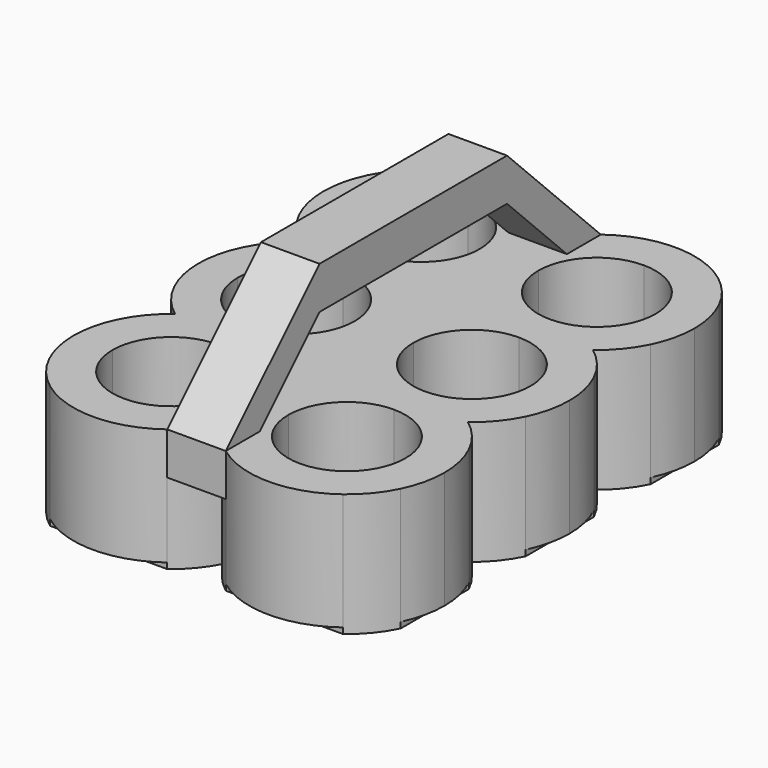
from build123d import *

# Parameters (mm, degrees)
F1_DEPTH = 25.4
F2_DEPTH = 1.27
F4_DEPTH = 6.35


with BuildPart() as f1:
    # F0 (on Top) → F1 (new body)
    with BuildSketch(Plane.XY):
        with BuildLine():
            Line((-2.1166666667, 33.8666666667), (-6.35, 33.8666666667))
            ThreePointArc((-6.35, 33.8666666667), (-10.0697438789, 24.8864105456), (-19.05, 21.1666666667))
            ThreePointArc((-19.05, 21.1666666667), (-12.356512286, 20.0804631421), (-6.35, 16.9333333333))
            ThreePointArc((-6.35, 16.9333333333), (-2.7139944723, 20.4069972362), (0, 24.6403305695))
            ThreePointArc((0, 24.6403305695), (-1.5807146965, 29.1336561143), (-2.1166666667, 33.8666666667))
        make_face()
        with BuildLine():
            ThreePointArc((-19.05, 46.5666666667), (-10.0697438789, 42.8469227877), (-6.35, 33.8666666667))
            Line((-6.35, 33.8666666667), (-2.1166666667, 33.8666666667))
            ThreePointArc((-2.1166666667, 33.8666666667), (-1.5807146965, 38.5996772191), (0, 43.0930027638))
            ThreePointArc((0, 43.0930027638), (-2.7139944723, 47.3263360972), (-6.35, 50.8))
            Line((-6.35, 50.8), (-19.05, 50.8))
            Line((-19.05, 50.8), (-19.05, 46.5666666667))
        make_face()
        with BuildLine():
            ThreePointArc((-31.75, 33.8666666667), (-28.0302561211, 42.8469227877), (-19.05, 46.5666666667))
            Line((-19.05, 46.5666666667), (-19.05, 50.8))
            Line((-19.05, 50.8), (-31.75, 50.8))
            ThreePointArc((-31.75, 50.8), (-35.3860055277, 47.3263360972), (-38.1, 43.0930027638))
            Line((-38.1, 43.0930027638), (-38.1, 33.8666666667))
            Line((-38.1, 33.8666666667), (-31.75, 33.8666666667))
        make_face()
        with BuildLine():
            ThreePointArc((-31.75, 16.9333333333), (-25.743487714, 20.0804631421), (-19.05, 21.1666666667))
            ThreePointArc((-19.05, 21.1666666667), (-28.0302561211, 24.8864105456), (-31.75, 33.8666666667))
            Line((-31.75, 33.8666666667), (-38.1, 33.8666666667))
            Line((-38.1, 33.8666666667), (-38.1, 24.6403305695))
            ThreePointArc((-38.1, 24.6403305695), (-35.3860055277, 20.4069972362), (-31.75, 16.9333333333))
        make_face()
        with BuildLine():
            ThreePointArc((-6.35, 16.9333333333), (-12.356512286, 20.0804631421), (-19.05, 21.1666666667))
            Line((-19.05, 21.1666666667), (-19.05, 16.9333333333))
            Line((-19.05, 16.9333333333), (-6.35, 16.9333333333))
        make_face()
        with BuildLine():
            Line((-19.05, 16.9333333333), (-19.05, 21.1666666667))
            ThreePointArc((-19.05, 21.1666666667), (-25.743487714, 20.0804631421), (-31.75, 16.9333333333))
            Line((-31.75, 16.9333333333), (-19.05, 16.9333333333))
        make_face()
        with BuildLine():
            ThreePointArc((0, 43.0930027638), (-1.5807146965, 38.5996772191), (-2.1166666667, 33.8666666667))
            Line((-2.1166666667, 33.8666666667), (0, 33.8666666667))
            Line((0, 33.8666666667), (0, 43.0930027638))
        make_face()
        with BuildLine():
            Line((0, 33.8666666667), (-2.1166666667, 33.8666666667))
            ThreePointArc((-2.1166666667, 33.8666666667), (-1.5807146965, 29.1336561143), (0, 24.6403305695))
            Line((0, 24.6403305695), (0, 33.8666666667))
        make_face()
        with BuildLine():
            Line((-31.75, 50.8), (-19.05, 50.8))
            Line((-19.05, 50.8), (-6.35, 50.8))
            ThreePointArc((-6.35, 50.8), (-19.05, 55.0333333333), (-31.75, 50.8))
        make_face()
        with BuildLine():
            Line((-6.35, 16.9333333333), (-19.05, 16.9333333333))
            Line((-19.05, 16.9333333333), (-19.05, 12.7))
            ThreePointArc((-19.0500000333, 12.7), (-12.3565123018, 13.7862035193), (-6.35, 16.9333333333))
        make_face()
        with BuildLine():
            Line((-19.05, 12.7), (-19.05, 16.9333333333))
            Line((-19.05, 16.9333333333), (-31.75, 16.9333333333))
            ThreePointArc((-31.75, 16.9333333333), (-25.7434877298, 13.7862035299), (-19.0500000333, 12.7))
        make_face()
        with BuildLine():
            ThreePointArc((0, 24.6403305695), (-2.7139944723, 20.4069972362), (-6.35, 16.9333333333))
            Line((-6.35, 16.9333333333), (0, 16.9333333333))
            Line((0, 16.9333333333), (0, 24.6403305695))
        make_face()
        with BuildLine():
            Line((0, 16.9333333333), (-6.35, 16.9333333333))
            ThreePointArc((-6.35, 16.9333333333), (-2.7139944723, 13.4596694305), (0, 9.2263360972))
            Line((0, 9.2263360972), (0, 16.9333333333))
        make_face()
        with BuildLine():
            ThreePointArc((0, 9.2263360972), (-2.7139944723, 13.4596694305), (-6.35, 16.9333333333))
            ThreePointArc((-6.35, 16.9333333333), (-12.3565123018, 13.7862035193), (-19.0500000333, 12.7))
            ThreePointArc((-19.0500000333, 12.7), (-10.0697438907, 8.9802561328), (-6.35, 0))
            Line((-6.35, 0), (-2.1166666667, 0))
            ThreePointArc((-2.1166666667, 0), (-1.5807146965, 4.7330105524), (0, 9.2263360972))
        make_face()
        with BuildLine():
            ThreePointArc((-19.0500000333, 12.7), (-25.7434877298, 13.7862035299), (-31.75, 16.9333333333))
            ThreePointArc((-31.75, 16.9333333333), (-35.3860055277, 13.4596694305), (-38.1, 9.2263360972))
            Line((-38.1, 9.2263360972), (-38.1, 0))
            Line((-38.1, 0), (-31.75, 0))
            ThreePointArc((-31.75, 0), (-28.0302561328, 8.9802561093), (-19.0500000333, 12.7))
        make_face()
        with BuildLine():
            Line((2.1166666667, 33.8666666667), (0, 33.8666666667))
            Line((0, 33.8666666667), (0, 24.6403305695))
            ThreePointArc((0, 24.6403305695), (1.5807146965, 29.1336561143), (2.1166666667, 33.8666666667))
        make_face()
        with BuildLine():
            Line((0, 43.0930027638), (0, 33.8666666667))
            Line((0, 33.8666666667), (2.1166666667, 33.8666666667))
            ThreePointArc((2.1166666667, 33.8666666667), (1.5807146965, 38.5996772191), (0, 43.0930027638))
        make_face()
        with BuildLine():
            ThreePointArc((6.35, 50.8), (2.7139944723, 47.3263360972), (0, 43.0930027638))
            ThreePointArc((0, 43.0930027638), (1.5807146965, 38.5996772191), (2.1166666667, 33.8666666667))
            Line((2.1166666667, 33.8666666667), (6.35, 33.8666666667))
            ThreePointArc((6.35, 33.8666666667), (10.0697438789, 42.8469227877), (19.05, 46.5666666667))
            Line((19.05, 46.5666666667), (19.05, 50.8))
            Line((19.05, 50.8), (6.35, 50.8))
        make_face()
        with BuildLine():
            ThreePointArc((6.35, 16.9333333333), (2.7139944723, 20.4069972362), (0, 24.6403305695))
            Line((0, 24.6403305695), (0, 16.9333333333))
            Line((0, 16.9333333333), (6.35, 16.9333333333))
        make_face()
        with BuildLine():
            ThreePointArc((2.1166666667, 33.8666666667), (1.5807146965, 29.1336561143), (0, 24.6403305695))
            ThreePointArc((0, 24.6403305695), (2.7139944723, 20.4069972362), (6.35, 16.9333333333))
            ThreePointArc((6.35, 16.9333333333), (12.356512286, 20.0804631421), (19.05, 21.1666666667))
            ThreePointArc((19.05, 21.1666666667), (10.0697438789, 24.8864105456), (6.35, 33.8666666667))
            Line((6.35, 33.8666666667), (2.1166666667, 33.8666666667))
        make_face()
        with BuildLine():
            Line((-38.1, 24.6403305695), (-38.1, 33.8666666667))
            Line((-38.1, 33.8666666667), (-38.1, 43.0930027638))
            ThreePointArc((-38.1, 43.0930027638), (-40.2166666667, 33.8666666667), (-38.1, 24.6403305695))
        make_face()
        with BuildLine():
            Line((6.35, 16.9333333333), (0, 16.9333333333))
            Line((0, 16.9333333333), (0, 9.2263360972))
            ThreePointArc((0, 9.2263360972), (2.7139944723, 13.4596694305), (6.35, 16.9333333333))
        make_face()
        with BuildLine():
            ThreePointArc((2.1166666667, 0), (1.5807146965, 4.7330105524), (0, 9.2263360972))
            Line((0, 9.2263360972), (0, 0))
            Line((0, 0), (2.1166666667, 0))
        make_face()
        with BuildLine():
            ThreePointArc((6.35, 16.9333333333), (2.7139944723, 13.4596694305), (0, 9.2263360972))
            ThreePointArc((0, 9.2263360972), (1.5807146965, 4.7330105524), (2.1166666667, 0))
            Line((2.1166666667, 0), (6.35, 0))
            ThreePointArc((6.35, 0), (10.0697438672, 8.9802561093), (19.0499999667, 12.7))
            ThreePointArc((19.0499999667, 12.7), (12.3565122702, 13.7862035299), (6.35, 16.9333333333))
        make_face()
        with BuildLine():
            Line((0, 0), (0, 9.2263360972))
            ThreePointArc((0, 9.2263360972), (-1.5807146965, 4.7330105524), (-2.1166666667, 0))
            Line((-2.1166666667, 0), (0, 0))
        make_face()
        with BuildLine():
            Line((-38.1, 0), (-38.1, 9.2263360972))
            ThreePointArc((-38.1, 9.2263360972), (-40.2166666667, 0), (-38.1, -9.2263360972))
            Line((-38.1, -9.2263360972), (-38.1, 0))
        make_face()
        with BuildLine():
            ThreePointArc((31.75, 50.8), (19.05, 55.0333333333), (6.35, 50.8))
            Line((6.35, 50.8), (19.05, 50.8))
            Line((19.05, 50.8), (31.75, 50.8))
        make_face()
        with BuildLine():
            ThreePointArc((19.05, 21.1666666667), (12.356512286, 20.0804631421), (6.35, 16.9333333333))
            Line((6.35, 16.9333333333), (19.05, 16.9333333333))
            Line((19.05, 16.9333333333), (19.05, 21.1666666667))
        make_face()
        with BuildLine():
            Line((19.05, 16.9333333333), (6.35, 16.9333333333))
            ThreePointArc((6.35, 16.9333333333), (12.3565122702, 13.7862035299), (19.0499999667, 12.7))
            Line((19.05, 12.7), (19.05, 16.9333333333))
        make_face()
        with BuildLine():
            Line((-2.1166666667, 0), (-6.35, 0))
            ThreePointArc((-6.35, 0), (-10.0697438789, -8.9802561211), (-19.05, -12.7))
            ThreePointArc((-19.05, -12.7), (-12.356512286, -13.7862035246), (-6.35, -16.9333333333))
            ThreePointArc((-6.35, -16.9333333333), (-2.7139944723, -13.4596694305), (0, -9.2263360972))
            ThreePointArc((0, -9.2263360972), (-1.5807146965, -4.7330105524), (-2.1166666667, 0))
        make_face()
        with BuildLine():
            ThreePointArc((-19.05, -12.7), (-28.0302561211, -8.9802561211), (-31.75, 0))
            Line((-31.75, 0), (-38.1, 0))
            Line((-38.1, 0), (-38.1, -9.2263360972))
            ThreePointArc((-38.1, -9.2263360972), (-35.3860055277, -13.4596694305), (-31.75, -16.9333333333))
            ThreePointArc((-31.75, -16.9333333333), (-25.743487714, -13.7862035246), (-19.05, -12.7))
        make_face()
        with BuildLine():
            Line((2.1166666667, 0), (0, 0))
            Line((0, 0), (0, -9.2263360972))
            ThreePointArc((0, -9.2263360972), (1.5807146965, -4.7330105524), (2.1166666667, 0))
        make_face()
        with BuildLine():
            Line((0, -9.2263360972), (0, 0))
            Line((0, 0), (-2.1166666667, 0))
            ThreePointArc((-2.1166666667, 0), (-1.5807146965, -4.7330105524), (0, -9.2263360972))
        make_face()
        with BuildLine():
            Line((6.35, 0), (2.1166666667, 0))
            ThreePointArc((2.1166666667, 0), (1.5807146965, -4.7330105524), (0, -9.2263360972))
            ThreePointArc((0, -9.2263360972), (2.7139944723, -13.4596694305), (6.35, -16.9333333333))
            ThreePointArc((6.35, -16.9333333333), (12.356512286, -13.7862035246), (19.05, -12.7))
            ThreePointArc((19.05, -12.7), (10.0697438789, -8.9802561211), (6.35, 0))
        make_face()
        with BuildLine():
            Line((31.75, 50.8), (19.05, 50.8))
            Line((19.05, 50.8), (19.05, 46.5666666667))
            ThreePointArc((19.05, 46.5666666667), (28.0302561211, 42.8469227877), (31.75, 33.8666666667))
            Line((31.75, 33.8666666667), (38.1, 33.8666666667))
            Line((38.1, 33.8666666667), (38.1, 43.0930027638))
            ThreePointArc((38.1, 43.0930027638), (35.3860055277, 47.3263360972), (31.75, 50.8))
        make_face()
        with BuildLine():
            Line((31.75, 16.9333333333), (19.05, 16.9333333333))
            Line((19.05, 16.9333333333), (19.05, 12.7))
            ThreePointArc((19.0499999667, 12.7), (25.7434876982, 13.7862035193), (31.75, 16.9333333333))
        make_face()
        with BuildLine():
            Line((19.05, 21.1666666667), (19.05, 16.9333333333))
            Line((19.05, 16.9333333333), (31.75, 16.9333333333))
            ThreePointArc((31.75, 16.9333333333), (25.743487714, 20.0804631421), (19.05, 21.1666666667))
        make_face()
        with BuildLine():
            ThreePointArc((31.75, 33.8666666667), (28.0302561211, 24.8864105456), (19.05, 21.1666666667))
            ThreePointArc((19.05, 21.1666666667), (25.743487714, 20.0804631421), (31.75, 16.9333333333))
            ThreePointArc((31.75, 16.9333333333), (35.3860055277, 20.4069972362), (38.1, 24.6403305695))
            Line((38.1, 24.6403305695), (38.1, 33.8666666667))
            Line((38.1, 33.8666666667), (31.75, 33.8666666667))
        make_face()
        with BuildLine():
            ThreePointArc((31.75, 16.9333333333), (25.7434876982, 13.7862035193), (19.0499999667, 12.7))
            ThreePointArc((19.0499999667, 12.7), (28.0302561093, 8.9802561328), (31.75, 0))
            Line((31.75, 0), (38.1, 0))
            Line((38.1, 0), (38.1, 9.2263360972))
            ThreePointArc((38.1, 9.2263360972), (35.3860055277, 13.4596694305), (31.75, 16.9333333333))
        make_face()
        with BuildLine():
            ThreePointArc((-6.35, -16.9333333333), (-12.356512286, -13.7862035246), (-19.05, -12.7))
            Line((-19.05, -12.7), (-19.05, -16.9333333333))
            Line((-19.05, -16.9333333333), (-6.35, -16.9333333333))
        make_face()
        with BuildLine():
            Line((-19.05, -16.9333333333), (-19.05, -12.7))
            ThreePointArc((-19.05, -12.7), (-25.743487714, -13.7862035246), (-31.75, -16.9333333333))
            Line((-31.75, -16.9333333333), (-19.05, -16.9333333333))
        make_face()
        with BuildLine():
            ThreePointArc((6.35, -16.9333333333), (2.7139944723, -13.4596694305), (0, -9.2263360972))
            Line((0, -9.2263360972), (0, -16.9333333333))
            Line((0, -16.9333333333), (6.35, -16.9333333333))
        make_face()
        with BuildLine():
            Line((0, -16.9333333333), (0, -9.2263360972))
            ThreePointArc((0, -9.2263360972), (-2.7139944723, -13.4596694305), (-6.35, -16.9333333333))
            Line((-6.35, -16.9333333333), (0, -16.9333333333))
        make_face()
        with BuildLine():
            Line((-19.05, -16.9333333333), (-31.75, -16.9333333333))
            ThreePointArc((-31.75, -16.9333333333), (-25.7434877142, -20.080463142), (-19.0500000004, -21.1666666667))
            Line((-19.05, -21.1666666667), (-19.05, -16.9333333333))
        make_face()
        with BuildLine():
            ThreePointArc((-19.0500000004, -21.1666666667), (-25.7434877142, -20.080463142), (-31.75, -16.9333333333))
            ThreePointArc((-31.75, -16.9333333333), (-35.3860055277, -20.4069972362), (-38.1, -24.6403305695))
            Line((-38.1, -24.6403305695), (-38.1, -33.8666666667))
            Line((-38.1, -33.8666666667), (-31.75, -33.8666666667))
            ThreePointArc((-31.75, -33.8666666667), (-28.0302561212, -24.8864105457), (-19.0500000004, -21.1666666667))
        make_face()
        with BuildLine():
            ThreePointArc((40.2166666667, 33.8666666667), (39.6807146965, 38.5996772191), (38.1, 43.0930027638))
            Line((38.1, 43.0930027638), (38.1, 33.8666666667))
            Line((38.1, 33.8666666667), (38.1, 24.6403305695))
            ThreePointArc((38.1, 24.6403305695), (39.6807146965, 29.1336561143), (40.2166666667, 33.8666666667))
        make_face()
        with BuildLine():
            Line((38.1, 0), (31.75, 0))
            ThreePointArc((31.75, 0), (28.0302561211, -8.9802561211), (19.05, -12.7))
            ThreePointArc((19.05, -12.7), (25.743487714, -13.7862035246), (31.75, -16.9333333333))
            ThreePointArc((31.75, -16.9333333333), (35.3860055277, -13.4596694305), (38.1, -9.2263360972))
            Line((38.1, -9.2263360972), (38.1, 0))
        make_face()
        with BuildLine():
            Line((-6.35, -16.9333333333), (-19.05, -16.9333333333))
            Line((-19.05, -16.9333333333), (-19.05, -21.1666666667))
            ThreePointArc((-19.0500000004, -21.1666666667), (-12.3565122862, -20.0804631421), (-6.35, -16.9333333333))
        make_face()
        with BuildLine():
            ThreePointArc((0, -24.6403305695), (-2.7139944723, -20.4069972362), (-6.35, -16.9333333333))
            ThreePointArc((-6.35, -16.9333333333), (-12.3565122862, -20.0804631421), (-19.0500000004, -21.1666666667))
            ThreePointArc((-19.0500000004, -21.1666666667), (-10.0697438791, -24.8864105455), (-6.35, -33.8666666667))
            Line((-6.35, -33.8666666667), (-2.1166666667, -33.8666666667))
            ThreePointArc((-2.1166666667, -33.8666666667), (-1.5807146965, -29.1336561143), (0, -24.6403305695))
        make_face()
        with BuildLine():
            Line((0, -16.9333333333), (-6.35, -16.9333333333))
            ThreePointArc((-6.35, -16.9333333333), (-2.7139944723, -20.4069972362), (0, -24.6403305695))
            Line((0, -24.6403305695), (0, -16.9333333333))
        make_face()
        with BuildLine():
            Line((6.35, -16.9333333333), (0, -16.9333333333))
            Line((0, -16.9333333333), (0, -24.6403305695))
            ThreePointArc((0, -24.6403305695), (2.7139944723, -20.4069972362), (6.35, -16.9333333333))
        make_face()
        with BuildLine():
            ThreePointArc((19.05, -12.7), (12.356512286, -13.7862035246), (6.35, -16.9333333333))
            Line((6.35, -16.9333333333), (19.05, -16.9333333333))
            Line((19.05, -16.9333333333), (19.05, -12.7))
        make_face()
        with BuildLine():
            Line((19.05, -16.9333333333), (6.35, -16.9333333333))
            ThreePointArc((6.35, -16.9333333333), (12.3565122858, -20.080463142), (19.0499999996, -21.1666666667))
            Line((19.05, -21.1666666667), (19.05, -16.9333333333))
        make_face()
        with BuildLine():
            ThreePointArc((19.0499999996, -21.1666666667), (12.3565122858, -20.080463142), (6.35, -16.9333333333))
            ThreePointArc((6.35, -16.9333333333), (2.7139944723, -20.4069972362), (0, -24.6403305695))
            ThreePointArc((0, -24.6403305695), (1.5807146965, -29.1336561143), (2.1166666667, -33.8666666667))
            Line((2.1166666667, -33.8666666667), (6.35, -33.8666666667))
            ThreePointArc((6.35, -33.8666666667), (10.0697438788, -24.8864105457), (19.0499999996, -21.1666666667))
        make_face()
        with BuildLine():
            ThreePointArc((31.75, -16.9333333333), (25.743487714, -13.7862035246), (19.05, -12.7))
            Line((19.05, -12.7), (19.05, -16.9333333333))
            Line((19.05, -16.9333333333), (31.75, -16.9333333333))
        make_face()
        with BuildLine():
            Line((-38.1, -33.8666666667), (-38.1, -24.6403305695))
            ThreePointArc((-38.1, -24.6403305695), (-40.2166666667, -33.8666666667), (-38.1, -43.0930027638))
            Line((-38.1, -43.0930027638), (-38.1, -33.8666666667))
        make_face()
        with BuildLine():
            ThreePointArc((40.2166666667, 0), (39.6807146965, 4.7330105524), (38.1, 9.2263360972))
            Line((38.1, 9.2263360972), (38.1, 0))
            Line((38.1, 0), (38.1, -9.2263360972))
            ThreePointArc((38.1, -9.2263360972), (39.6807146965, -4.7330105524), (40.2166666667, 0))
        make_face()
        with BuildLine():
            ThreePointArc((2.1166666667, -33.8666666667), (1.5807146965, -29.1336561143), (0, -24.6403305695))
            Line((0, -24.6403305695), (0, -33.8666666667))
            Line((0, -33.8666666667), (2.1166666667, -33.8666666667))
        make_face()
        with BuildLine():
            Line((0, -33.8666666667), (0, -24.6403305695))
            ThreePointArc((0, -24.6403305695), (-1.5807146965, -29.1336561143), (-2.1166666667, -33.8666666667))
            Line((-2.1166666667, -33.8666666667), (0, -33.8666666667))
        make_face()
        with BuildLine():
            Line((31.75, -16.9333333333), (19.05, -16.9333333333))
            Line((19.05, -16.9333333333), (19.05, -21.1666666667))
            ThreePointArc((19.0499999996, -21.1666666667), (25.7434877138, -20.0804631421), (31.75, -16.9333333333))
        make_face()
        with BuildLine():
            ThreePointArc((31.75, -16.9333333333), (25.7434877138, -20.0804631421), (19.0499999996, -21.1666666667))
            ThreePointArc((19.0499999996, -21.1666666667), (28.0302561209, -24.8864105455), (31.75, -33.8666666667))
            Line((31.75, -33.8666666667), (38.1, -33.8666666667))
            Line((38.1, -33.8666666667), (38.1, -24.6403305695))
            ThreePointArc((38.1, -24.6403305695), (35.3860055277, -20.4069972362), (31.75, -16.9333333333))
        make_face()
        with BuildLine():
            Line((-31.75, -33.8666666667), (-38.1, -33.8666666667))
            Line((-38.1, -33.8666666667), (-38.1, -43.0930027638))
            ThreePointArc((-38.1, -43.0930027638), (-35.3860055276, -47.3263360972), (-31.75, -50.8))
            Line((-31.75, -50.8), (-19.05, -50.8))
            Line((-19.05, -50.8), (-19.05, -46.5666666667))
            ThreePointArc((-19.05, -46.5666666667), (-28.0302561211, -42.8469227877), (-31.75, -33.8666666667))
        make_face()
        with BuildLine():
            Line((-2.1166666667, -33.8666666667), (-6.35, -33.8666666667))
            ThreePointArc((-6.35, -33.8666666667), (-10.0697438789, -42.8469227877), (-19.05, -46.5666666667))
            Line((-19.05, -46.5666666667), (-19.05, -50.8))
            Line((-19.05, -50.8), (-6.35, -50.8))
            ThreePointArc((-6.35, -50.8), (-2.7139944724, -47.3263360971), (0, -43.0930027638))
            ThreePointArc((0, -43.0930027638), (-1.5807146965, -38.599677219), (-2.1166666667, -33.8666666667))
        make_face()
        with BuildLine():
            Line((2.1166666667, -33.8666666667), (0, -33.8666666667))
            Line((0, -33.8666666667), (0, -43.0930027638))
            ThreePointArc((0, -43.0930027638), (1.5807146965, -38.599677219), (2.1166666667, -33.8666666667))
        make_face()
        with BuildLine():
            Line((0, -43.0930027638), (0, -33.8666666667))
            Line((0, -33.8666666667), (-2.1166666667, -33.8666666667))
            ThreePointArc((-2.1166666667, -33.8666666667), (-1.5807146965, -38.599677219), (0, -43.0930027638))
        make_face()
        with BuildLine():
            Line((6.35, -33.8666666667), (2.1166666667, -33.8666666667))
            ThreePointArc((2.1166666667, -33.8666666667), (1.5807146965, -38.599677219), (0, -43.0930027638))
            ThreePointArc((0, -43.0930027638), (2.7139944724, -47.3263360972), (6.35, -50.8))
            Line((6.35, -50.8), (19.05, -50.8))
            Line((19.05, -50.8), (19.05, -46.5666666667))
            ThreePointArc((19.05, -46.5666666667), (10.0697438789, -42.8469227877), (6.35, -33.8666666667))
        make_face()
        with BuildLine():
            Line((38.1, -33.8666666667), (31.75, -33.8666666667))
            ThreePointArc((31.75, -33.8666666667), (28.0302561211, -42.8469227877), (19.05, -46.5666666667))
            Line((19.05, -46.5666666667), (19.05, -50.8))
            Line((19.05, -50.8), (31.75, -50.8))
            ThreePointArc((31.75, -50.8), (35.3860055276, -47.3263360971), (38.1, -43.0930027638))
            Line((38.1, -43.0930027638), (38.1, -33.8666666667))
        make_face()
        with BuildLine():
            ThreePointArc((40.2166666667, -33.8666666667), (39.6807146965, -29.1336561143), (38.1, -24.6403305695))
            Line((38.1, -24.6403305695), (38.1, -33.8666666667))
            Line((38.1, -33.8666666667), (38.1, -43.0930027638))
            ThreePointArc((38.1, -43.0930027638), (39.6807146965, -38.599677219), (40.2166666667, -33.8666666667))
        make_face()
        with BuildLine():
            Line((-19.05, -50.8), (-31.75, -50.8))
            ThreePointArc((-31.75, -50.8), (-19.05, -55.0333333333), (-6.35, -50.8))
            Line((-6.35, -50.8), (-19.05, -50.8))
        make_face()
        with BuildLine():
            Line((19.05, -50.8), (6.35, -50.8))
            ThreePointArc((6.35, -50.8), (19.05, -55.0333333333), (31.75, -50.8))
            Line((31.75, -50.8), (19.05, -50.8))
        make_face()
    extrude(amount=F1_DEPTH)

    # F0 (on Top) → F2 (join, symmetric)
    with BuildSketch(Plane.XY):
        with BuildLine():
            Line((-19.05, 33.8666666667), (-19.05, 46.5666666667))
            ThreePointArc((-19.05, 46.5666666667), (-28.0302561211, 42.8469227877), (-31.75, 33.8666666667))
            Line((-31.75, 33.8666666667), (-19.05, 33.8666666667))
        make_face()
        with BuildLine():
            Line((-19.05, 33.8666666667), (-6.35, 33.8666666667))
            ThreePointArc((-6.35, 33.8666666667), (-10.0697438789, 42.8469227877), (-19.05, 46.5666666667))
            Line((-19.05, 46.5666666667), (-19.05, 33.8666666667))
        make_face()
        with BuildLine():
            ThreePointArc((-31.75, 33.8666666667), (-28.0302561211, 24.8864105456), (-19.05, 21.1666666667))
            Line((-19.05, 21.1666666667), (-19.05, 33.8666666667))
            Line((-19.05, 33.8666666667), (-31.75, 33.8666666667))
        make_face()
        with BuildLine():
            ThreePointArc((-19.05, 21.1666666667), (-10.0697438789, 24.8864105456), (-6.35, 33.8666666667))
            Line((-6.35, 33.8666666667), (-19.05, 33.8666666667))
            Line((-19.05, 33.8666666667), (-19.05, 21.1666666667))
        make_face()
        with BuildLine():
            ThreePointArc((19.05, 46.5666666667), (10.0697438789, 42.8469227877), (6.35, 33.8666666667))
            Line((6.35, 33.8666666667), (19.05, 33.8666666667))
            Line((19.05, 33.8666666667), (19.05, 46.5666666667))
        make_face()
        with BuildLine():
            ThreePointArc((31.75, 33.8666666667), (28.0302561211, 42.8469227877), (19.05, 46.5666666667))
            Line((19.05, 46.5666666667), (19.05, 33.8666666667))
            Line((19.05, 33.8666666667), (31.75, 33.8666666667))
        make_face()
        with BuildLine():
            Line((19.05, 33.8666666667), (19.05, 21.1666666667))
            ThreePointArc((19.05, 21.1666666667), (28.0302561211, 24.8864105456), (31.75, 33.8666666667))
            Line((31.75, 33.8666666667), (19.05, 33.8666666667))
        make_face()
        with BuildLine():
            Line((19.05, 33.8666666667), (6.35, 33.8666666667))
            ThreePointArc((6.35, 33.8666666667), (10.0697438789, 24.8864105456), (19.05, 21.1666666667))
            Line((19.05, 21.1666666667), (19.05, 33.8666666667))
        make_face()
        with BuildLine():
            Line((-19.05, 0), (-19.05, 12.7))
            ThreePointArc((-19.0500000333, 12.7), (-28.0302561328, 8.9802561093), (-31.75, 0))
            Line((-31.75, 0), (-19.05, 0))
        make_face()
        with BuildLine():
            ThreePointArc((-6.35, 0), (-10.0697438907, 8.9802561328), (-19.0500000333, 12.7))
            Line((-19.05, 12.7), (-19.05, 0))
            Line((-19.05, 0), (-6.35, 0))
        make_face()
        with BuildLine():
            Line((-19.05, 0), (-31.75, 0))
            ThreePointArc((-31.75, 0), (-28.0302561211, -8.9802561211), (-19.05, -12.7))
            Line((-19.05, -12.7), (-19.05, 0))
        make_face()
        with BuildLine():
            ThreePointArc((-19.05, -12.7), (-10.0697438789, -8.9802561211), (-6.35, 0))
            Line((-6.35, 0), (-19.05, 0))
            Line((-19.05, 0), (-19.05, -12.7))
        make_face()
        with BuildLine():
            Line((19.05, 0), (19.05, 12.7))
            ThreePointArc((19.0499999667, 12.7), (10.0697438672, 8.9802561093), (6.35, 0))
            Line((6.35, 0), (19.05, 0))
        make_face()
        with BuildLine():
            Line((19.05, 0), (6.35, 0))
            ThreePointArc((6.35, 0), (10.0697438789, -8.9802561211), (19.05, -12.7))
            Line((19.05, -12.7), (19.05, 0))
        make_face()
        with BuildLine():
            ThreePointArc((19.05, -12.7), (28.0302561211, -8.9802561211), (31.75, 0))
            Line((31.75, 0), (19.05, 0))
            Line((19.05, 0), (19.05, -12.7))
        make_face()
        with BuildLine():
            ThreePointArc((31.75, 0), (28.0302561093, 8.9802561328), (19.0499999667, 12.7))
            Line((19.05, 12.7), (19.05, 0))
            Line((19.05, 0), (31.75, 0))
        make_face()
        with BuildLine():
            ThreePointArc((-6.35, -33.8666666667), (-10.0697438791, -24.8864105455), (-19.0500000004, -21.1666666667))
            Line((-19.05, -21.1666666667), (-19.05, -33.8666666667))
            Line((-19.05, -33.8666666667), (-6.35, -33.8666666667))
        make_face()
        with BuildLine():
            Line((-19.05, -33.8666666667), (-19.05, -21.1666666667))
            ThreePointArc((-19.0500000004, -21.1666666667), (-28.0302561212, -24.8864105457), (-31.75, -33.8666666667))
            Line((-31.75, -33.8666666667), (-19.05, -33.8666666667))
        make_face()
        with BuildLine():
            Line((-19.05, -33.8666666667), (-31.75, -33.8666666667))
            ThreePointArc((-31.75, -33.8666666667), (-28.0302561211, -42.8469227877), (-19.05, -46.5666666667))
            Line((-19.05, -46.5666666667), (-19.05, -33.8666666667))
        make_face()
        with BuildLine():
            ThreePointArc((-19.05, -46.5666666667), (-10.0697438789, -42.8469227877), (-6.35, -33.8666666667))
            Line((-6.35, -33.8666666667), (-19.05, -33.8666666667))
            Line((-19.05, -33.8666666667), (-19.05, -46.5666666667))
        make_face()
        with BuildLine():
            Line((19.05, -33.8666666667), (19.05, -21.1666666667))
            ThreePointArc((19.0499999996, -21.1666666667), (10.0697438788, -24.8864105457), (6.35, -33.8666666667))
            Line((6.35, -33.8666666667), (19.05, -33.8666666667))
        make_face()
        with BuildLine():
            Line((19.05, -33.8666666667), (6.35, -33.8666666667))
            ThreePointArc((6.35, -33.8666666667), (10.0697438789, -42.8469227877), (19.05, -46.5666666667))
            Line((19.05, -46.5666666667), (19.05, -33.8666666667))
        make_face()
        with BuildLine():
            ThreePointArc((19.05, -46.5666666667), (28.0302561211, -42.8469227877), (31.75, -33.8666666667))
            Line((31.75, -33.8666666667), (19.05, -33.8666666667))
            Line((19.05, -33.8666666667), (19.05, -46.5666666667))
        make_face()
        with BuildLine():
            ThreePointArc((31.75, -33.8666666667), (28.0302561209, -24.8864105455), (19.0499999996, -21.1666666667))
            Line((19.05, -21.1666666667), (19.05, -33.8666666667))
            Line((19.05, -33.8666666667), (31.75, -33.8666666667))
        make_face()
        with BuildLine():
            Line((19.05, -16.9333333333), (6.35, -16.9333333333))
            ThreePointArc((6.35, -16.9333333333), (12.3565122858, -20.080463142), (19.0499999996, -21.1666666667))
            Line((19.05, -21.1666666667), (19.05, -16.9333333333))
        make_face()
        with BuildLine():
            Line((31.75, -16.9333333333), (19.05, -16.9333333333))
            Line((19.05, -16.9333333333), (19.05, -21.1666666667))
            ThreePointArc((19.0499999996, -21.1666666667), (25.7434877138, -20.0804631421), (31.75, -16.9333333333))
        make_face()
        with BuildLine():
            ThreePointArc((31.75, -16.9333333333), (25.743487714, -13.7862035246), (19.05, -12.7))
            Line((19.05, -12.7), (19.05, -16.9333333333))
            Line((19.05, -16.9333333333), (31.75, -16.9333333333))
        make_face()
        with BuildLine():
            ThreePointArc((19.05, -12.7), (12.356512286, -13.7862035246), (6.35, -16.9333333333))
            Line((6.35, -16.9333333333), (19.05, -16.9333333333))
            Line((19.05, -16.9333333333), (19.05, -12.7))
        make_face()
        with BuildLine():
            ThreePointArc((-6.35, -16.9333333333), (-12.356512286, -13.7862035246), (-19.05, -12.7))
            Line((-19.05, -12.7), (-19.05, -16.9333333333))
            Line((-19.05, -16.9333333333), (-6.35, -16.9333333333))
        make_face()
        with BuildLine():
            Line((-6.35, -16.9333333333), (-19.05, -16.9333333333))
            Line((-19.05, -16.9333333333), (-19.05, -21.1666666667))
            ThreePointArc((-19.0500000004, -21.1666666667), (-12.3565122862, -20.0804631421), (-6.35, -16.9333333333))
        make_face()
        with BuildLine():
            Line((-19.05, -16.9333333333), (-31.75, -16.9333333333))
            ThreePointArc((-31.75, -16.9333333333), (-25.7434877142, -20.080463142), (-19.0500000004, -21.1666666667))
            Line((-19.05, -21.1666666667), (-19.05, -16.9333333333))
        make_face()
        with BuildLine():
            Line((-19.05, -16.9333333333), (-19.05, -12.7))
            ThreePointArc((-19.05, -12.7), (-25.743487714, -13.7862035246), (-31.75, -16.9333333333))
            Line((-31.75, -16.9333333333), (-19.05, -16.9333333333))
        make_face()
        with BuildLine():
            Line((-19.05, 16.9333333333), (-19.05, 21.1666666667))
            ThreePointArc((-19.05, 21.1666666667), (-25.743487714, 20.0804631421), (-31.75, 16.9333333333))
            Line((-31.75, 16.9333333333), (-19.05, 16.9333333333))
        make_face()
        with BuildLine():
            Line((-19.05, 12.7), (-19.05, 16.9333333333))
            Line((-19.05, 16.9333333333), (-31.75, 16.9333333333))
            ThreePointArc((-31.75, 16.9333333333), (-25.7434877298, 13.7862035299), (-19.0500000333, 12.7))
        make_face()
        with BuildLine():
            Line((-6.35, 16.9333333333), (-19.05, 16.9333333333))
            Line((-19.05, 16.9333333333), (-19.05, 12.7))
            ThreePointArc((-19.0500000333, 12.7), (-12.3565123018, 13.7862035193), (-6.35, 16.9333333333))
        make_face()
        with BuildLine():
            ThreePointArc((-6.35, 16.9333333333), (-12.356512286, 20.0804631421), (-19.05, 21.1666666667))
            Line((-19.05, 21.1666666667), (-19.05, 16.9333333333))
            Line((-19.05, 16.9333333333), (-6.35, 16.9333333333))
        make_face()
        with BuildLine():
            ThreePointArc((19.05, 21.1666666667), (12.356512286, 20.0804631421), (6.35, 16.9333333333))
            Line((6.35, 16.9333333333), (19.05, 16.9333333333))
            Line((19.05, 16.9333333333), (19.05, 21.1666666667))
        make_face()
        with BuildLine():
            Line((19.05, 16.9333333333), (6.35, 16.9333333333))
            ThreePointArc((6.35, 16.9333333333), (12.3565122702, 13.7862035299), (19.0499999667, 12.7))
            Line((19.05, 12.7), (19.05, 16.9333333333))
        make_face()
        with BuildLine():
            Line((31.75, 16.9333333333), (19.05, 16.9333333333))
            Line((19.05, 16.9333333333), (19.05, 12.7))
            ThreePointArc((19.0499999667, 12.7), (25.7434876982, 13.7862035193), (31.75, 16.9333333333))
        make_face()
        with BuildLine():
            Line((19.05, 21.1666666667), (19.05, 16.9333333333))
            Line((19.05, 16.9333333333), (31.75, 16.9333333333))
            ThreePointArc((31.75, 16.9333333333), (25.743487714, 20.0804631421), (19.05, 21.1666666667))
        make_face()
        with BuildLine():
            Line((2.1166666667, 33.8666666667), (0, 33.8666666667))
            Line((0, 33.8666666667), (0, 24.6403305695))
            ThreePointArc((0, 24.6403305695), (1.5807146965, 29.1336561143), (2.1166666667, 33.8666666667))
        make_face()
        with BuildLine():
            Line((0, 33.8666666667), (-2.1166666667, 33.8666666667))
            ThreePointArc((-2.1166666667, 33.8666666667), (-1.5807146965, 29.1336561143), (0, 24.6403305695))
            Line((0, 24.6403305695), (0, 33.8666666667))
        make_face()
        with BuildLine():
            ThreePointArc((0, 43.0930027638), (-1.5807146965, 38.5996772191), (-2.1166666667, 33.8666666667))
            Line((-2.1166666667, 33.8666666667), (0, 33.8666666667))
            Line((0, 33.8666666667), (0, 43.0930027638))
        make_face()
        with BuildLine():
            Line((0, 43.0930027638), (0, 33.8666666667))
            Line((0, 33.8666666667), (2.1166666667, 33.8666666667))
            ThreePointArc((2.1166666667, 33.8666666667), (1.5807146965, 38.5996772191), (0, 43.0930027638))
        make_face()
        with BuildLine():
            ThreePointArc((-19.05, 46.5666666667), (-10.0697438789, 42.8469227877), (-6.35, 33.8666666667))
            Line((-6.35, 33.8666666667), (-2.1166666667, 33.8666666667))
            ThreePointArc((-2.1166666667, 33.8666666667), (-1.5807146965, 38.5996772191), (0, 43.0930027638))
            ThreePointArc((0, 43.0930027638), (-2.7139944723, 47.3263360972), (-6.35, 50.8))
            Line((-6.35, 50.8), (-19.05, 50.8))
            Line((-19.05, 50.8), (-19.05, 46.5666666667))
        make_face()
        with BuildLine():
            Line((-2.1166666667, 33.8666666667), (-6.35, 33.8666666667))
            ThreePointArc((-6.35, 33.8666666667), (-10.0697438789, 24.8864105456), (-19.05, 21.1666666667))
            ThreePointArc((-19.05, 21.1666666667), (-12.356512286, 20.0804631421), (-6.35, 16.9333333333))
            ThreePointArc((-6.35, 16.9333333333), (-2.7139944723, 20.4069972362), (0, 24.6403305695))
            ThreePointArc((0, 24.6403305695), (-1.5807146965, 29.1336561143), (-2.1166666667, 33.8666666667))
        make_face()
        with BuildLine():
            ThreePointArc((2.1166666667, 33.8666666667), (1.5807146965, 29.1336561143), (0, 24.6403305695))
            ThreePointArc((0, 24.6403305695), (2.7139944723, 20.4069972362), (6.35, 16.9333333333))
            ThreePointArc((6.35, 16.9333333333), (12.356512286, 20.0804631421), (19.05, 21.1666666667))
            ThreePointArc((19.05, 21.1666666667), (10.0697438789, 24.8864105456), (6.35, 33.8666666667))
            Line((6.35, 33.8666666667), (2.1166666667, 33.8666666667))
        make_face()
        with BuildLine():
            ThreePointArc((6.35, 50.8), (2.7139944723, 47.3263360972), (0, 43.0930027638))
            ThreePointArc((0, 43.0930027638), (1.5807146965, 38.5996772191), (2.1166666667, 33.8666666667))
            Line((2.1166666667, 33.8666666667), (6.35, 33.8666666667))
            ThreePointArc((6.35, 33.8666666667), (10.0697438789, 42.8469227877), (19.05, 46.5666666667))
            Line((19.05, 46.5666666667), (19.05, 50.8))
            Line((19.05, 50.8), (6.35, 50.8))
        make_face()
        with BuildLine():
            ThreePointArc((0, 9.2263360972), (-2.7139944723, 13.4596694305), (-6.35, 16.9333333333))
            ThreePointArc((-6.35, 16.9333333333), (-12.3565123018, 13.7862035193), (-19.0500000333, 12.7))
            ThreePointArc((-19.0500000333, 12.7), (-10.0697438907, 8.9802561328), (-6.35, 0))
            Line((-6.35, 0), (-2.1166666667, 0))
            ThreePointArc((-2.1166666667, 0), (-1.5807146965, 4.7330105524), (0, 9.2263360972))
        make_face()
        with BuildLine():
            ThreePointArc((6.35, 16.9333333333), (2.7139944723, 13.4596694305), (0, 9.2263360972))
            ThreePointArc((0, 9.2263360972), (1.5807146965, 4.7330105524), (2.1166666667, 0))
            Line((2.1166666667, 0), (6.35, 0))
            ThreePointArc((6.35, 0), (10.0697438672, 8.9802561093), (19.0499999667, 12.7))
            ThreePointArc((19.0499999667, 12.7), (12.3565122702, 13.7862035299), (6.35, 16.9333333333))
        make_face()
        with BuildLine():
            Line((0, 0), (0, 9.2263360972))
            ThreePointArc((0, 9.2263360972), (-1.5807146965, 4.7330105524), (-2.1166666667, 0))
            Line((-2.1166666667, 0), (0, 0))
        make_face()
        with BuildLine():
            Line((2.1166666667, 0), (0, 0))
            Line((0, 0), (0, -9.2263360972))
            ThreePointArc((0, -9.2263360972), (1.5807146965, -4.7330105524), (2.1166666667, 0))
        make_face()
        with BuildLine():
            Line((0, -9.2263360972), (0, 0))
            Line((0, 0), (-2.1166666667, 0))
            ThreePointArc((-2.1166666667, 0), (-1.5807146965, -4.7330105524), (0, -9.2263360972))
        make_face()
        with BuildLine():
            ThreePointArc((2.1166666667, 0), (1.5807146965, 4.7330105524), (0, 9.2263360972))
            Line((0, 9.2263360972), (0, 0))
            Line((0, 0), (2.1166666667, 0))
        make_face()
        with BuildLine():
            Line((6.35, 0), (2.1166666667, 0))
            ThreePointArc((2.1166666667, 0), (1.5807146965, -4.7330105524), (0, -9.2263360972))
            ThreePointArc((0, -9.2263360972), (2.7139944723, -13.4596694305), (6.35, -16.9333333333))
            ThreePointArc((6.35, -16.9333333333), (12.356512286, -13.7862035246), (19.05, -12.7))
            ThreePointArc((19.05, -12.7), (10.0697438789, -8.9802561211), (6.35, 0))
        make_face()
        with BuildLine():
            Line((-2.1166666667, 0), (-6.35, 0))
            ThreePointArc((-6.35, 0), (-10.0697438789, -8.9802561211), (-19.05, -12.7))
            ThreePointArc((-19.05, -12.7), (-12.356512286, -13.7862035246), (-6.35, -16.9333333333))
            ThreePointArc((-6.35, -16.9333333333), (-2.7139944723, -13.4596694305), (0, -9.2263360972))
            ThreePointArc((0, -9.2263360972), (-1.5807146965, -4.7330105524), (-2.1166666667, 0))
        make_face()
        with BuildLine():
            ThreePointArc((0, -24.6403305695), (-2.7139944723, -20.4069972362), (-6.35, -16.9333333333))
            ThreePointArc((-6.35, -16.9333333333), (-12.3565122862, -20.0804631421), (-19.0500000004, -21.1666666667))
            ThreePointArc((-19.0500000004, -21.1666666667), (-10.0697438791, -24.8864105455), (-6.35, -33.8666666667))
            Line((-6.35, -33.8666666667), (-2.1166666667, -33.8666666667))
            ThreePointArc((-2.1166666667, -33.8666666667), (-1.5807146965, -29.1336561143), (0, -24.6403305695))
        make_face()
        with BuildLine():
            Line((-2.1166666667, -33.8666666667), (-6.35, -33.8666666667))
            ThreePointArc((-6.35, -33.8666666667), (-10.0697438789, -42.8469227877), (-19.05, -46.5666666667))
            Line((-19.05, -46.5666666667), (-19.05, -50.8))
            Line((-19.05, -50.8), (-6.35, -50.8))
            ThreePointArc((-6.35, -50.8), (-2.7139944724, -47.3263360971), (0, -43.0930027638))
            ThreePointArc((0, -43.0930027638), (-1.5807146965, -38.599677219), (-2.1166666667, -33.8666666667))
        make_face()
        with BuildLine():
            Line((0, -43.0930027638), (0, -33.8666666667))
            Line((0, -33.8666666667), (-2.1166666667, -33.8666666667))
            ThreePointArc((-2.1166666667, -33.8666666667), (-1.5807146965, -38.599677219), (0, -43.0930027638))
        make_face()
        with BuildLine():
            Line((6.35, -33.8666666667), (2.1166666667, -33.8666666667))
            ThreePointArc((2.1166666667, -33.8666666667), (1.5807146965, -38.599677219), (0, -43.0930027638))
            ThreePointArc((0, -43.0930027638), (2.7139944724, -47.3263360972), (6.35, -50.8))
            Line((6.35, -50.8), (19.05, -50.8))
            Line((19.05, -50.8), (19.05, -46.5666666667))
            ThreePointArc((19.05, -46.5666666667), (10.0697438789, -42.8469227877), (6.35, -33.8666666667))
        make_face()
        with BuildLine():
            ThreePointArc((2.1166666667, -33.8666666667), (1.5807146965, -29.1336561143), (0, -24.6403305695))
            Line((0, -24.6403305695), (0, -33.8666666667))
            Line((0, -33.8666666667), (2.1166666667, -33.8666666667))
        make_face()
        with BuildLine():
            Line((0, -33.8666666667), (0, -24.6403305695))
            ThreePointArc((0, -24.6403305695), (-1.5807146965, -29.1336561143), (-2.1166666667, -33.8666666667))
            Line((-2.1166666667, -33.8666666667), (0, -33.8666666667))
        make_face()
        with BuildLine():
            ThreePointArc((19.0499999996, -21.1666666667), (12.3565122858, -20.080463142), (6.35, -16.9333333333))
            ThreePointArc((6.35, -16.9333333333), (2.7139944723, -20.4069972362), (0, -24.6403305695))
            ThreePointArc((0, -24.6403305695), (1.5807146965, -29.1336561143), (2.1166666667, -33.8666666667))
            Line((2.1166666667, -33.8666666667), (6.35, -33.8666666667))
            ThreePointArc((6.35, -33.8666666667), (10.0697438788, -24.8864105457), (19.0499999996, -21.1666666667))
        make_face()
        with BuildLine():
            Line((2.1166666667, -33.8666666667), (0, -33.8666666667))
            Line((0, -33.8666666667), (0, -43.0930027638))
            ThreePointArc((0, -43.0930027638), (1.5807146965, -38.599677219), (2.1166666667, -33.8666666667))
        make_face()
        with BuildLine():
            Line((0, 16.9333333333), (-6.35, 16.9333333333))
            ThreePointArc((-6.35, 16.9333333333), (-2.7139944723, 13.4596694305), (0, 9.2263360972))
            Line((0, 9.2263360972), (0, 16.9333333333))
        make_face()
        with BuildLine():
            Line((6.35, 16.9333333333), (0, 16.9333333333))
            Line((0, 16.9333333333), (0, 9.2263360972))
            ThreePointArc((0, 9.2263360972), (2.7139944723, 13.4596694305), (6.35, 16.9333333333))
        make_face()
        with BuildLine():
            ThreePointArc((0, 24.6403305695), (-2.7139944723, 20.4069972362), (-6.35, 16.9333333333))
            Line((-6.35, 16.9333333333), (0, 16.9333333333))
            Line((0, 16.9333333333), (0, 24.6403305695))
        make_face()
        with BuildLine():
            Line((0, -16.9333333333), (0, -9.2263360972))
            ThreePointArc((0, -9.2263360972), (-2.7139944723, -13.4596694305), (-6.35, -16.9333333333))
            Line((-6.35, -16.9333333333), (0, -16.9333333333))
        make_face()
        with BuildLine():
            ThreePointArc((6.35, -16.9333333333), (2.7139944723, -13.4596694305), (0, -9.2263360972))
            Line((0, -9.2263360972), (0, -16.9333333333))
            Line((0, -16.9333333333), (6.35, -16.9333333333))
        make_face()
        with BuildLine():
            Line((0, -16.9333333333), (-6.35, -16.9333333333))
            ThreePointArc((-6.35, -16.9333333333), (-2.7139944723, -20.4069972362), (0, -24.6403305695))
            Line((0, -24.6403305695), (0, -16.9333333333))
        make_face()
        with BuildLine():
            Line((6.35, -16.9333333333), (0, -16.9333333333))
            Line((0, -16.9333333333), (0, -24.6403305695))
            ThreePointArc((0, -24.6403305695), (2.7139944723, -20.4069972362), (6.35, -16.9333333333))
        make_face()
        with BuildLine():
            ThreePointArc((6.35, 16.9333333333), (2.7139944723, 20.4069972362), (0, 24.6403305695))
            Line((0, 24.6403305695), (0, 16.9333333333))
            Line((0, 16.9333333333), (6.35, 16.9333333333))
        make_face()
        with BuildLine():
            ThreePointArc((-19.0500000333, 12.7), (-25.7434877298, 13.7862035299), (-31.75, 16.9333333333))
            ThreePointArc((-31.75, 16.9333333333), (-35.3860055277, 13.4596694305), (-38.1, 9.2263360972))
            Line((-38.1, 9.2263360972), (-38.1, 0))
            Line((-38.1, 0), (-31.75, 0))
            ThreePointArc((-31.75, 0), (-28.0302561328, 8.9802561093), (-19.0500000333, 12.7))
        make_face()
        with BuildLine():
            ThreePointArc((-19.05, -12.7), (-28.0302561211, -8.9802561211), (-31.75, 0))
            Line((-31.75, 0), (-38.1, 0))
            Line((-38.1, 0), (-38.1, -9.2263360972))
            ThreePointArc((-38.1, -9.2263360972), (-35.3860055277, -13.4596694305), (-31.75, -16.9333333333))
            ThreePointArc((-31.75, -16.9333333333), (-25.743487714, -13.7862035246), (-19.05, -12.7))
        make_face()
        with BuildLine():
            ThreePointArc((-31.75, 16.9333333333), (-25.743487714, 20.0804631421), (-19.05, 21.1666666667))
            ThreePointArc((-19.05, 21.1666666667), (-28.0302561211, 24.8864105456), (-31.75, 33.8666666667))
            Line((-31.75, 33.8666666667), (-38.1, 33.8666666667))
            Line((-38.1, 33.8666666667), (-38.1, 24.6403305695))
            ThreePointArc((-38.1, 24.6403305695), (-35.3860055277, 20.4069972362), (-31.75, 16.9333333333))
        make_face()
        with BuildLine():
            ThreePointArc((-31.75, 33.8666666667), (-28.0302561211, 42.8469227877), (-19.05, 46.5666666667))
            Line((-19.05, 46.5666666667), (-19.05, 50.8))
            Line((-19.05, 50.8), (-31.75, 50.8))
            ThreePointArc((-31.75, 50.8), (-35.3860055277, 47.3263360972), (-38.1, 43.0930027638))
            Line((-38.1, 43.0930027638), (-38.1, 33.8666666667))
            Line((-38.1, 33.8666666667), (-31.75, 33.8666666667))
        make_face()
        with BuildLine():
            Line((31.75, 50.8), (19.05, 50.8))
            Line((19.05, 50.8), (19.05, 46.5666666667))
            ThreePointArc((19.05, 46.5666666667), (28.0302561211, 42.8469227877), (31.75, 33.8666666667))
            Line((31.75, 33.8666666667), (38.1, 33.8666666667))
            Line((38.1, 33.8666666667), (38.1, 43.0930027638))
            ThreePointArc((38.1, 43.0930027638), (35.3860055277, 47.3263360972), (31.75, 50.8))
        make_face()
        with BuildLine():
            ThreePointArc((31.75, 33.8666666667), (28.0302561211, 24.8864105456), (19.05, 21.1666666667))
            ThreePointArc((19.05, 21.1666666667), (25.743487714, 20.0804631421), (31.75, 16.9333333333))
            ThreePointArc((31.75, 16.9333333333), (35.3860055277, 20.4069972362), (38.1, 24.6403305695))
            Line((38.1, 24.6403305695), (38.1, 33.8666666667))
            Line((38.1, 33.8666666667), (31.75, 33.8666666667))
        make_face()
        with BuildLine():
            ThreePointArc((31.75, 16.9333333333), (25.7434876982, 13.7862035193), (19.0499999667, 12.7))
            ThreePointArc((19.0499999667, 12.7), (28.0302561093, 8.9802561328), (31.75, 0))
            Line((31.75, 0), (38.1, 0))
            Line((38.1, 0), (38.1, 9.2263360972))
            ThreePointArc((38.1, 9.2263360972), (35.3860055277, 13.4596694305), (31.75, 16.9333333333))
        make_face()
        with BuildLine():
            Line((38.1, 0), (31.75, 0))
            ThreePointArc((31.75, 0), (28.0302561211, -8.9802561211), (19.05, -12.7))
            ThreePointArc((19.05, -12.7), (25.743487714, -13.7862035246), (31.75, -16.9333333333))
            ThreePointArc((31.75, -16.9333333333), (35.3860055277, -13.4596694305), (38.1, -9.2263360972))
            Line((38.1, -9.2263360972), (38.1, 0))
        make_face()
        with BuildLine():
            ThreePointArc((31.75, -16.9333333333), (25.7434877138, -20.0804631421), (19.0499999996, -21.1666666667))
            ThreePointArc((19.0499999996, -21.1666666667), (28.0302561209, -24.8864105455), (31.75, -33.8666666667))
            Line((31.75, -33.8666666667), (38.1, -33.8666666667))
            Line((38.1, -33.8666666667), (38.1, -24.6403305695))
            ThreePointArc((38.1, -24.6403305695), (35.3860055277, -20.4069972362), (31.75, -16.9333333333))
        make_face()
        with BuildLine():
            Line((38.1, -33.8666666667), (31.75, -33.8666666667))
            ThreePointArc((31.75, -33.8666666667), (28.0302561211, -42.8469227877), (19.05, -46.5666666667))
            Line((19.05, -46.5666666667), (19.05, -50.8))
            Line((19.05, -50.8), (31.75, -50.8))
            ThreePointArc((31.75, -50.8), (35.3860055276, -47.3263360971), (38.1, -43.0930027638))
            Line((38.1, -43.0930027638), (38.1, -33.8666666667))
        make_face()
        with BuildLine():
            Line((-31.75, -33.8666666667), (-38.1, -33.8666666667))
            Line((-38.1, -33.8666666667), (-38.1, -43.0930027638))
            ThreePointArc((-38.1, -43.0930027638), (-35.3860055276, -47.3263360972), (-31.75, -50.8))
            Line((-31.75, -50.8), (-19.05, -50.8))
            Line((-19.05, -50.8), (-19.05, -46.5666666667))
            ThreePointArc((-19.05, -46.5666666667), (-28.0302561211, -42.8469227877), (-31.75, -33.8666666667))
        make_face()
        with BuildLine():
            ThreePointArc((-19.0500000004, -21.1666666667), (-25.7434877142, -20.080463142), (-31.75, -16.9333333333))
            ThreePointArc((-31.75, -16.9333333333), (-35.3860055277, -20.4069972362), (-38.1, -24.6403305695))
            Line((-38.1, -24.6403305695), (-38.1, -33.8666666667))
            Line((-38.1, -33.8666666667), (-31.75, -33.8666666667))
            ThreePointArc((-31.75, -33.8666666667), (-28.0302561212, -24.8864105457), (-19.0500000004, -21.1666666667))
        make_face()
    extrude(amount=F2_DEPTH, both=True)

    # F3 (on Right) → F4 (join, symmetric)
    with BuildSketch(Plane.YZ):
        Polygon((0, 50.8), (0, 41.6108981431), (25.4, 41.6108981431), (50.8, 16.2108981431), (50.8, 25.4), (25.4, 50.8), align=None)
        Polygon((-25.4, 41.6108981431), (0, 41.6108981431), (0, 50.8), (-25.4, 50.8), (-50.8, 25.4), (-50.8, 16.2108981431), align=None)
    extrude(amount=F4_DEPTH, both=True)


solid = f1.part
